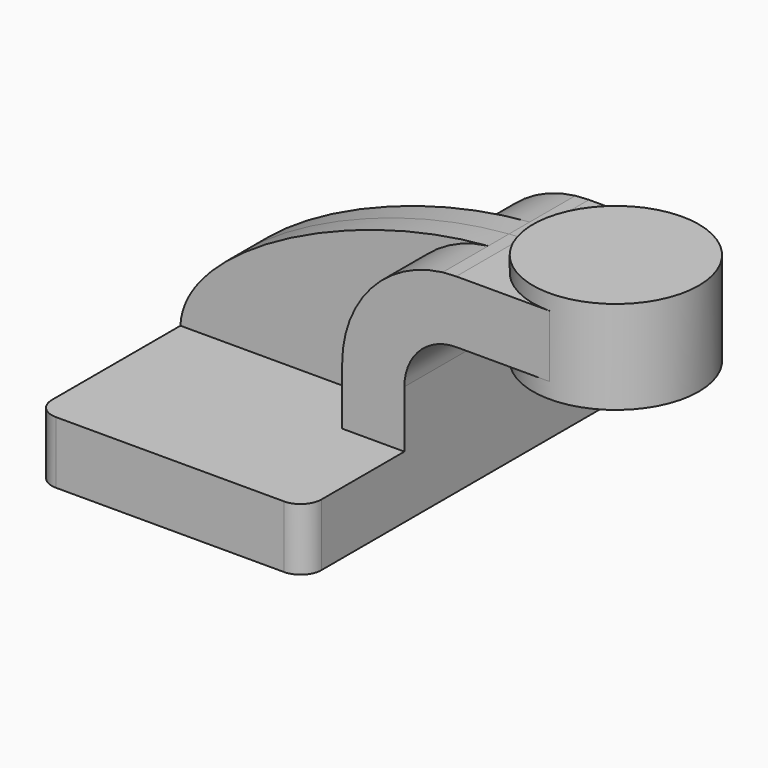
from build123d import *

# Parameters (mm, degrees)
F1_DEPTH = 63.5
F0_W     = 25.4
F0_H     = 19.05
F2_DEPTH = 25.4
F3_DEPTH = 7.9375
F5_R     = 6.35


# Not quite as in the source:
# - a feature names something its author has since deleted; it is built from what else it names


with BuildPart() as f1:
    # F0 (on Front) → F1 (new body, symmetric)
    with BuildSketch(Plane.XZ):
        Polygon((41.275, -9.525), (41.275, 9.525), (22.225, 9.525), (-41.275, 9.525), (-41.275, -9.525), align=None)
    extrude(amount=F1_DEPTH, both=True)

    # F0 (on Front) → F2 (join, symmetric)
    with BuildSketch(Plane.XZ):
        with BuildLine():
            Line((22.225, 9.525), (41.275, 9.525))
            Line((41.275, 9.525), (41.275, 27.0003691794))
            ThreePointArc((41.275, 27.0003691794), (45.8987977719, 38.19974744), (57.0767100375, 42.8752))
            Line((57.0767100375, 42.8752), (60.325, 42.8752))
            Line((60.325, 42.8752), (60.325, 61.9252))
            Line((60.325, 61.9252), (57.15, 61.9252))
            add(Edge.make_bspline(
                [(52.9909613243, 61.6768456771), (54.385845827, 61.7839036656), (55.7728431111, 61.8669849), (57.15, 61.9252)],
                knots=[107.9985895846, 107.9985895846, 107.9985895846, 107.9985895846, 111.5045361635, 111.5045361635, 111.5045361635, 111.5045361635], degree=3))
            ThreePointArc((52.9909613243, 61.6768456771), (31.0252028644, 50.1790360873), (22.225, 27.0003691794))
            Line((22.225, 27.0003691794), (22.225, 9.525))
        make_face()
        with Locations((73.025, 52.4002)):
            Rectangle(F0_W, F0_H)
    extrude(amount=F2_DEPTH, both=True)

    # F0 (on Front) → F3 (join, symmetric)
    with BuildSketch(Plane.XZ):
        with BuildLine():
            Line((-41.275, 9.525), (22.225, 9.525))
            Line((22.225, 9.525), (22.225, 27.0003691794))
            ThreePointArc((22.225, 27.0003691794), (31.0252028644, 50.1790360873), (52.9909613243, 61.6768456771))
            add(Edge.make_bspline(
                [(-41.275, 9.525), (-40.4304762971, 32.3293201332), (10.0223776518, 58.3789883087), (52.9909613243, 61.6768456771)],
                knots=[0, 0, 0, 0, 107.9985895846, 107.9985895846, 107.9985895846, 107.9985895846], degree=3))
        make_face()
    extrude(amount=F3_DEPTH, both=True)

    # F0 (on Front) → F4 (revolve)
    with BuildSketch(Plane.XZ):
        Polygon((85.725, 61.9252), (85.725, 42.8752), (85.725, 38.1), (111.125, 38.1), (111.125, 66.675), (85.725, 66.675), align=None)
    revolve(axis=Axis((85.725, 0, 52.3875), (0, 0, 1)))

    # F5
    f5_edges = [f1.edges().sort_by_distance(p)[0] for p in [
        (41.275, -63.5, 0),
        (-41.275, -63.5, 0),
        (41.275, 63.5, 0),
        (-41.275, 63.5, 0),
    ]]
    fillet(f5_edges, radius=F5_R)


solid = f1.part
